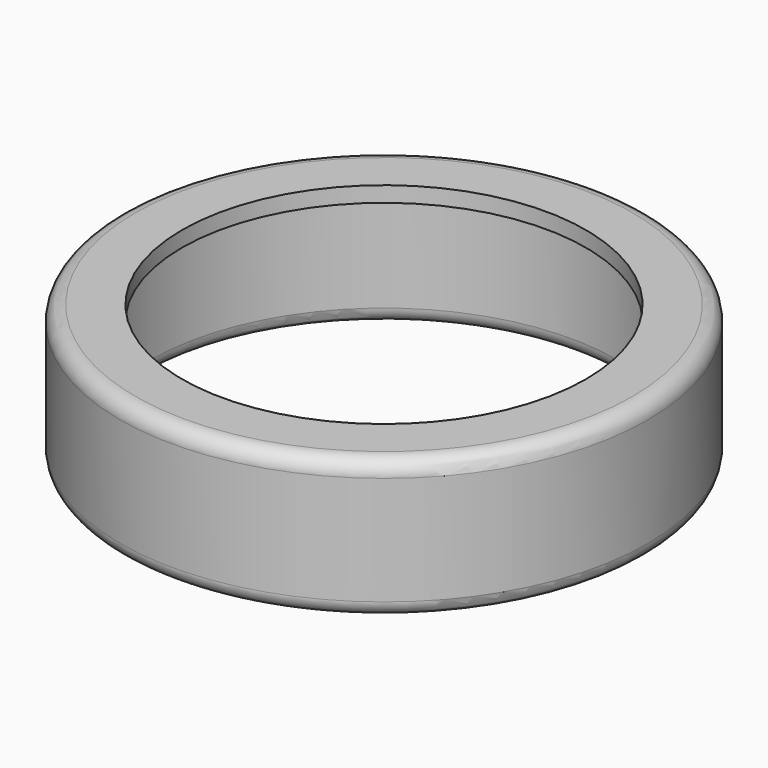
from build123d import *

# Parameters (mm, degrees)
F0_R     = 17
F1_DEPTH = 8
F2_R     = 15
F3_DEPTH = 8
F4_R     = 17
F5_DEPTH = 1
F6_R     = 13
F7_DEPTH = 1
F8_R     = 0.99999
F9_R     = 1


# Not quite as in the source:
# - a fillet or chamfer is up to 0.001 mm smaller than in the source, because OpenCascade refuses the exact size


with BuildPart() as f1:
    # F0 (on Top) → F1 (new body)
    with BuildSketch(Plane.XY):
        Circle(F0_R)
    extrude(amount=F1_DEPTH)

    # F2 (on face) → F3 (cut)
    with BuildSketch(Plane(origin=(0, 0, 0), x_dir=(1, 0, 0), z_dir=(0, 0, -1))):
        Circle(F2_R)
    extrude(amount=-F3_DEPTH, mode=Mode.SUBTRACT)

    # F4 (on face) → F5 (join)
    with BuildSketch(Plane.XY.offset(8)):
        Circle(F4_R)
    extrude(amount=F5_DEPTH)

    # F6 (on face) → F7 (cut)
    with BuildSketch(Plane.XY.offset(9)):
        Circle(F6_R)
    extrude(amount=-F7_DEPTH, mode=Mode.SUBTRACT)

    # F8 (radius 1 in the source; OpenCascade refuses exactly that, so slightly less here)
    f8_edges = [f1.edges().sort_by_distance(p)[0] for p in [
        (-17, 0, 0),
        (-15, 0, 0),
    ]]
    fillet(f8_edges, radius=F8_R)

    # F9
    f9_edges = [f1.edges().sort_by_distance(p)[0] for p in [
        (-17, 0, 9),
    ]]
    fillet(f9_edges, radius=F9_R)


solid = f1.part
